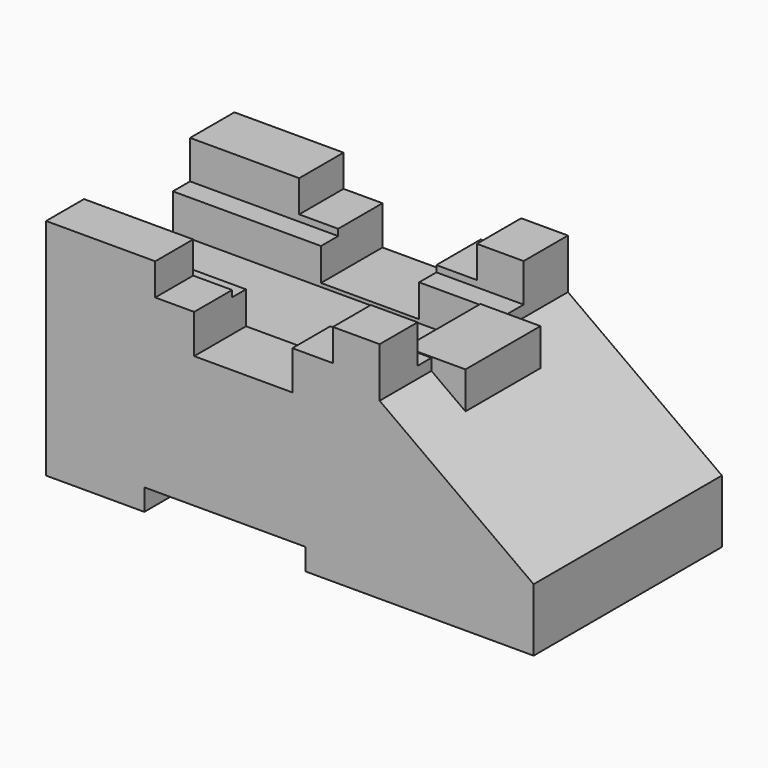
from build123d import *

# Parameters (mm, degrees)
F0_W      = 43.5
F0_H      = 20
F1_DEPTH  = 21
F2_W      = 23.5
F2_H      = 2
F3_DEPTH  = 79
F4_W      = 8.7595684454
F4_H      = 3.4760199487
F4_W_2    = 14.3907200545
F4_H_2    = 1.9311879296
F5_DEPTH  = 21.001
F6_W      = 18.0619247258
F6_H      = 11.0779828392
F7_DEPTH  = 20.001
F8_W      = 8.364611771
F8_H      = 3.2224319875
F9_DEPTH  = 43.501
F10_DEPTH = 13.8
F11_DEPTH = 16.0159093717
F12_W     = 5.3562937983
F12_H     = 8.364611771
F13_DEPTH = 3.3


# Not quite as in the source:
# - an extrude ends at something that could not be found from the text; its depth is read off the source's solid


with BuildPart() as f1:
    # F0 (on Front) → F1 (new body)
    with BuildSketch(Plane.XZ):
        with Locations((21.75, 10)):
            Rectangle(F0_W, F0_H)
    extrude(amount=F1_DEPTH)

    # F2 (on Front) → F3 (cut, through all)
    with BuildSketch(Plane.XZ):
        with Locations((15.8696506918, 1)):
            Rectangle(F2_W, F2_H)
    extrude(amount=-F3_DEPTH, mode=Mode.SUBTRACT)

    # F4 (on face) → F5 (cut, through all)
    with BuildSketch(Plane.XZ.offset(21)):
        Polygon((25.5898274481, 20), (9.7391782328, 20), (9.7391782328, 17.1561539173), (13.2151981816, 17.1561539173), (21.974766627, 17.1561539173), (25.5898274481, 17.1561539173), align=None)
        with Locations((17.5949824043, 15.418143943)):
            Rectangle(F4_W, F4_H)
        with Locations((15.9612530842, 0.9655939648)):
            Rectangle(F4_W_2, F4_H_2)
        Polygon((43.5, 20), (29.7610498965, 20), (29.7610498965, 15.5571838841), (43.5, 5.6157684885), align=None)
    extrude(amount=-F5_DEPTH, mode=Mode.SUBTRACT)

    # F6 (on Top) → F7 (cut, through all)
    with BuildSketch(Plane.XY):
        with Locations((38.8933513314, -10.4759179521)):
            Rectangle(F6_W, F6_H)
    extrude(amount=F7_DEPTH, mode=Mode.SUBTRACT)

    # F8 (on face) → F9 (cut, through all)
    with BuildSketch(Plane(origin=(0, 0, 0), x_dir=(0, -1, 0), z_dir=(-1, 0, 0))):
        with Locations((11.04275533, 14.9709172547)):
            Rectangle(F8_W, F8_H)
        Polygon((16.7677160352, 20), (4.9407021143, 20), (4.9407021143, 16.5821332484), (6.8604494445, 16.5821332484), (15.2250612155, 16.5821332484), (16.7677160352, 16.5821332484), align=None)
    extrude(amount=-F9_DEPTH, mode=Mode.SUBTRACT)

    # F10 (add): a face of the model
    f10_faces = [f1.faces().sort_by_distance(p)[0] for p in [
        (29.8623889685, -10.4104180179, 6.9700489552),
    ]]
    extrude(f10_faces, amount=F10_DEPTH)

    # F11 (cut, through all): a face of the model
    f11_faces = [f1.faces().sort_by_distance(p)[0] for p in [
        (39.1208034391, -16.0149093717, 12.034105167),
    ]]
    extrude(f11_faces, amount=-F11_DEPTH, mode=Mode.SUBTRACT)

    # F12 (on face) → F13 (join)
    with BuildSketch(Plane.XY.offset(13.3597012609)):
        with Locations((30.1198049788, -11.04275533)):
            Rectangle(F12_W, F12_H)
    extrude(amount=F13_DEPTH)


solid = f1.part
